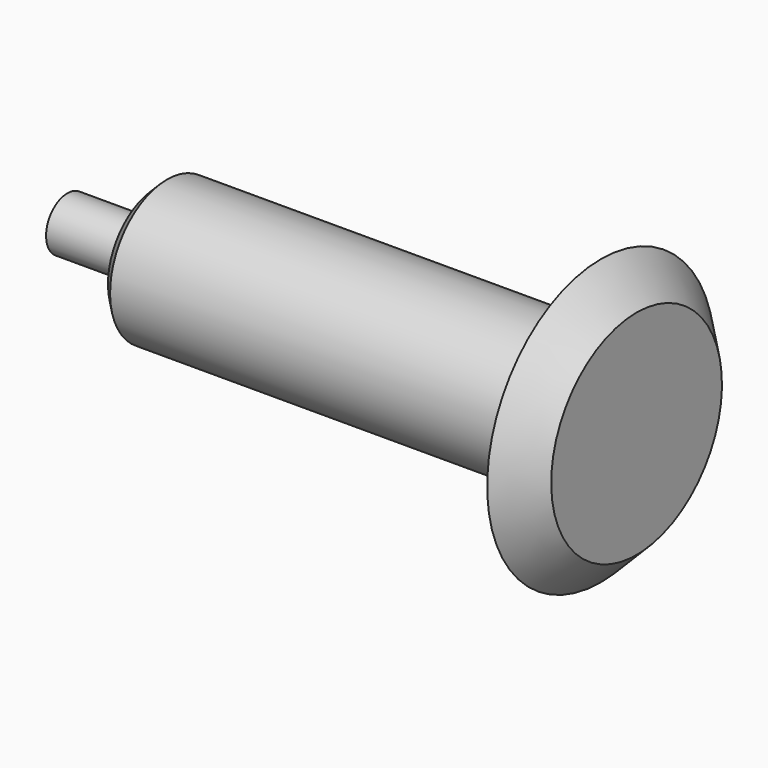
from build123d import *

# Parameters (mm, degrees)
F2_SIZE2 = 3
F2_SIZE  = 3
F3_SIZE2 = 10
F3_SIZE  = 10
F4_SIZE2 = 9.99999
F4_SIZE  = 9.99999


# Not quite as in the source:
# - a fillet or chamfer is up to 0.001 mm smaller than in the source, because OpenCascade refuses the exact size


with BuildPart() as f1:
    # F0 (on Front) → F1 (revolve)
    with BuildSketch(Plane.XZ):
        Polygon((0, 7.5), (0, 0), (160, 0), (160, 40), (150, 40), (150, 20), (25, 20), (25, 7.5), align=None)
    revolve(axis=Axis((80, 0, 0), (-1, 0, 0)))

    # F2
    f2_edges = [f1.edges().sort_by_distance(p)[0] for p in [
        (25, 0, -20),
    ]]
    chamfer(f2_edges, length=F2_SIZE, length2=F2_SIZE2)

    # F3
    f3_edges = [f1.edges().sort_by_distance(p)[0] for p in [
        (150, 0, -20),
    ]]
    chamfer(f3_edges, length=F3_SIZE, length2=F3_SIZE2)

    # F4 (size 10 and 10 in the source; OpenCascade refuses exactly that, so slightly less here)
    f4_edges = [f1.edges().sort_by_distance(p)[0] for p in [
        (160, 0, -40),
    ]]
    chamfer(f4_edges, length=F4_SIZE, length2=F4_SIZE2)


solid = f1.part
